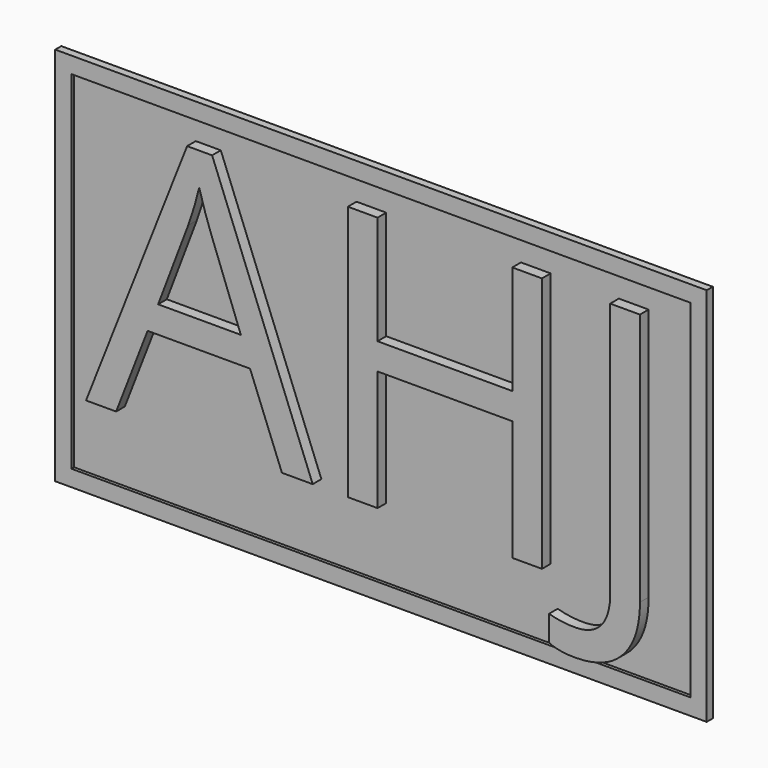
from build123d import *

# Parameters (mm, degrees)
F0_W         = 600
F0_H         = 350
F0_W_2       = 570
F0_H_2       = 320
F1_DEPTH     = 7
F2_DEPTH     = 4
F3_W         = 320
F3_H         = 220
F4_DEPTH     = 20
F5_R         = 10
F6_DEPTH     = 10
F7_TEXT_SIZE = 329.8807889223
F8_DEPTH     = 10


# Not quite as in the source:
# - Text() gives the source's letters only with a copy of the font that has no kerning and outlines rounded to 1/6400 em; it was checked with that copy


with BuildPart() as f1:
    # F0 (on Front) → F1 (new body)
    with BuildSketch(Plane.XZ):
        Rectangle(F0_W, F0_H)
        Rectangle(F0_W_2, F0_H_2, mode=Mode.SUBTRACT)
    extrude(amount=F1_DEPTH)

    # F0 (on Front) → F2 (join)
    with BuildSketch(Plane.XZ):
        Rectangle(F0_W_2, F0_H_2)
    extrude(amount=F2_DEPTH)

    # F3 (on face) → F4 (join)
    with BuildSketch(Plane.XZ):
        Rectangle(F3_W, F3_H)
    extrude(amount=-F4_DEPTH)

    # F5 (on face) → F6 (cut)
    with BuildSketch(Plane(origin=(0, 20, 0), x_dir=(-1, 0, 0), z_dir=(0, 1, 0))):
        Circle(F5_R)
    extrude(amount=-F6_DEPTH, mode=Mode.SUBTRACT)

    # F7 (on face) → F8 (join)
    with BuildSketch(Plane.XZ.offset(4)):
        with Locations((-266.0283987061, -95.5696925521)):
            Text('AHJ', F7_TEXT_SIZE, font='Open Sans', text_align=(TextAlign.LEFT, TextAlign.BOTTOM))
    extrude(amount=F8_DEPTH)


solid = f1.part
